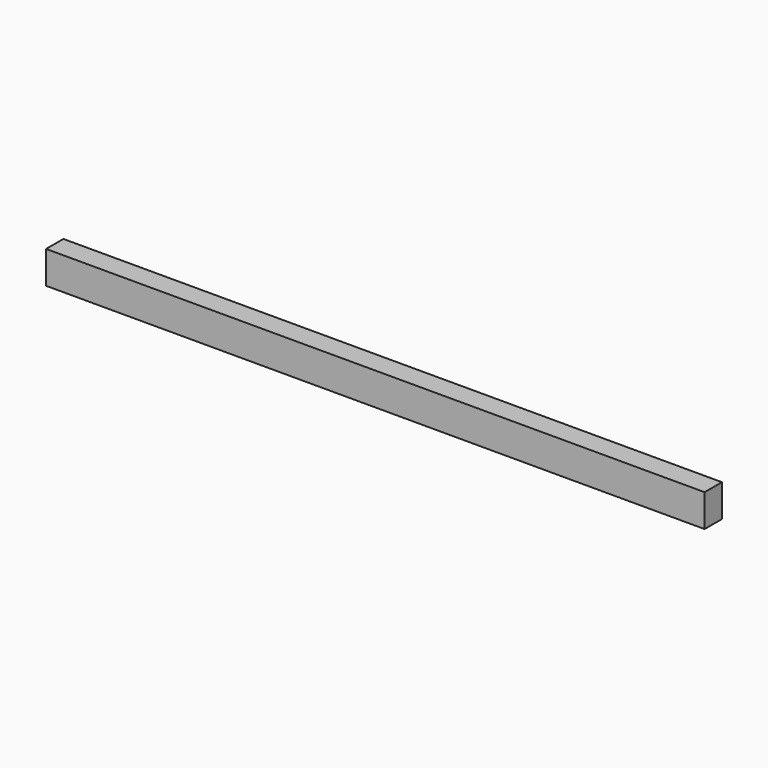
from build123d import *

# Parameters (mm, degrees)
F0_W     = 386.08
F0_H     = 19.05
F1_DEPTH = 12.7


# Not quite as in the source:
# - a feature names something its author has since deleted; it is built from what else it names


with BuildPart() as f1:
    # F0 (on Front) → F1 (new body)
    with BuildSketch(Plane.XZ):
        with Locations((132.0800510788, 144.9867119074)):
            Rectangle(F0_W, F0_H)
    extrude(amount=F1_DEPTH)


solid = f1.part
